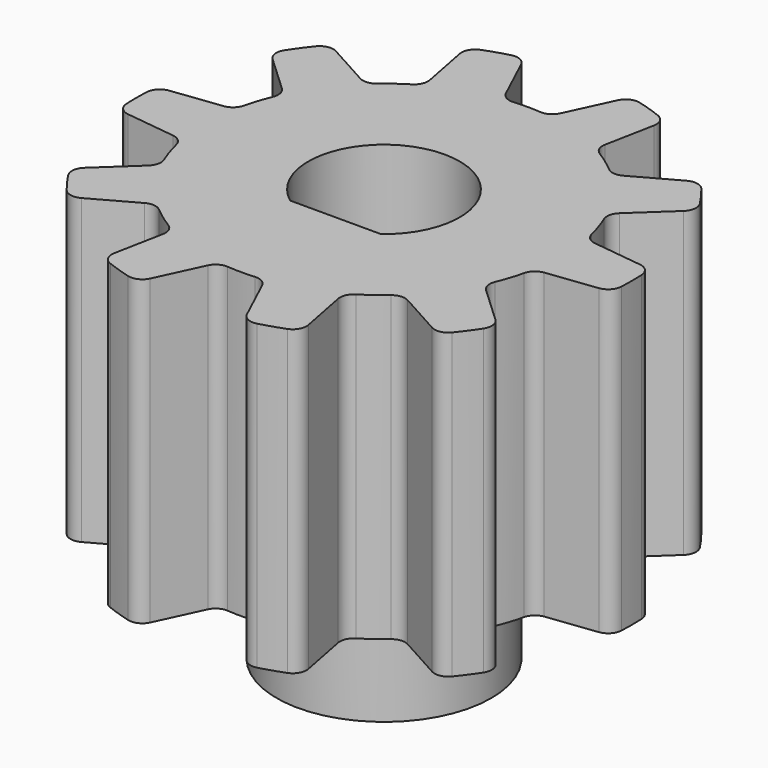
from build123d import *

# Parameters (mm, degrees)
F0_W            = 9
F0_H            = 11
F3_DEPTH        = 12
F3_COPIES_COUNT = 10
F5_DEPTH        = 25
F6_R            = 3.9
F7_DEPTH        = 4


# Not quite as in the source:
# - a pattern or mirror of a feature is missing from the dataset's text; its kind, count and spacing are read off the source's solid


with BuildPart() as f1:
    # F0 (on Front) → F1 (revolve)
    with BuildSketch(Plane.XZ):
        with Locations((-4.5, 5.5)):
            Rectangle(F0_W, F0_H)
    revolve(axis=Axis((0, 0, 5.5), (0, 0, 1)))

    # F2 (on face) → F3 (cut)
    with BuildSketch(Plane.XY.offset(11)):
        with BuildLine():
            ThreePointArc((-0.495692908, 6.4810715581), (0, 6.5), (0.495692908, 6.4810715581))
            ThreePointArc((0.495692908, 6.4810715581), (0.7861862119, 6.5479757718), (0.9869770252, 6.7683063932))
            Line((0.9869770252, 6.7683063932), (1.7567161864, 8.4190173512))
            ThreePointArc((1.7567161864, 8.4190173512), (1.9988344627, 8.6609895549), (2.3398624375, 8.6905145862))
            ThreePointArc((2.3398624375, 8.6905145862), (0, 9), (-2.3398624375, 8.6905145862))
            ThreePointArc((-2.3398624375, 8.6905145862), (-1.9988344627, 8.6609895549), (-1.7567161864, 8.4190173512))
            Line((-1.7567161864, 8.4190173512), (-0.9869770252, 6.7683063932))
            ThreePointArc((-0.9869770252, 6.7683063932), (-0.7861862119, 6.5479757718), (-0.495692908, 6.4810715581))
        make_face()
    f3 = extrude(amount=-F3_DEPTH, mode=Mode.SUBTRACT)

    # F3_copies: F3 ×10 about axis
    f3_copies_axis = Axis((0, 0, 0), (0, 0, 1))
    for i in range(1, F3_COPIES_COUNT):
        add(f3.rotate(f3_copies_axis, i * 360 / F3_COPIES_COUNT), mode=Mode.SUBTRACT)

    # F4 (on face) → F5 (cut)
    with BuildSketch(Plane.XY.offset(11)):
        with BuildLine():
            Line((-1.65, -2.2), (1.65, -2.2))
            ThreePointArc((1.65, -2.2), (0, 2.75), (-1.65, -2.2))
        make_face()
    extrude(amount=-F5_DEPTH, mode=Mode.SUBTRACT)

    # F6 (on face) → F7 (join)
    with BuildSketch(Plane(origin=(0, 0, 0), x_dir=(1, 0, 0), z_dir=(0, 0, -1))):
        Circle(F6_R)
        with BuildLine():
            ThreePointArc((1.65, 2.2), (0, -2.75), (-1.65, 2.2))
            Line((-1.65, 2.2), (1.65, 2.2))
        make_face(mode=Mode.SUBTRACT)
    extrude(amount=F7_DEPTH)


solid = f1.part
